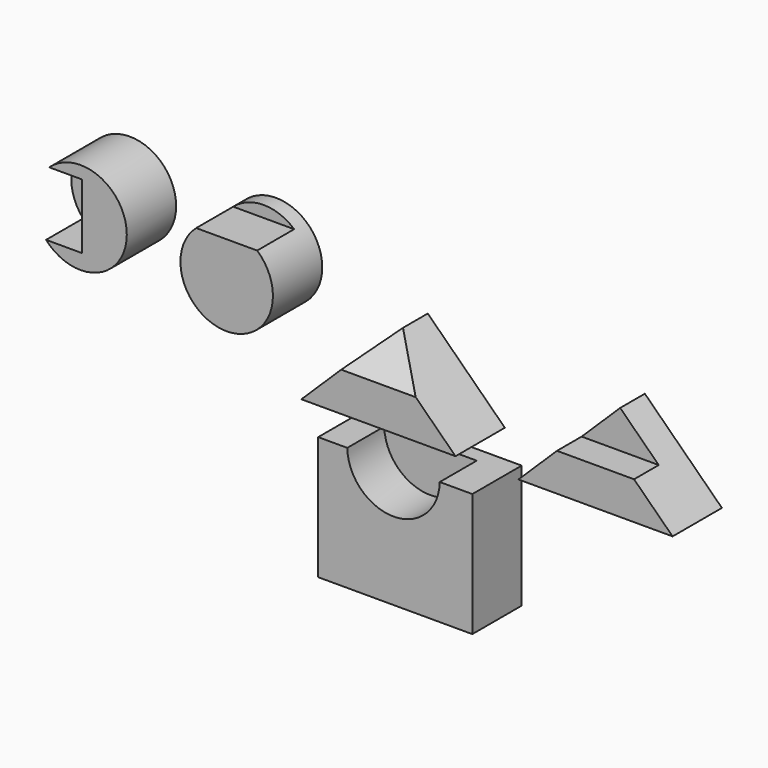
from build123d import *

# Parameters (mm, degrees)
F1_DEPTH  = 101.6
F2_DEPTH  = 50.8
F4_DEPTH  = 101.6
F8_DEPTH  = 63.5
F9_R      = 76.2
F10_DEPTH = 101.6
F11_W     = 138.8424634933
F11_H     = 72.9273408651
F12_DEPTH = 76.2
F13_R     = 76.2
F14_DEPTH = 101.6
F15_W     = 160.2847576141
F15_H     = 106.856547296
F16_DEPTH = 76.2
F17_W     = 254
F17_H     = 203.2
F18_DEPTH = 101.6
F19_R     = 76.2
F20_DEPTH = 76.2


with BuildPart() as f1:
    # F0 (on Front) → F1 (new body)
    with BuildSketch(Plane.XZ):
        Polygon((63.5, 62.2170394667), (0, 0), (254, 0), (190.5, 62.2170394667), align=None)
    extrude(amount=F1_DEPTH)

    # F0 (on Front) → F2 (join)
    with BuildSketch(Plane.XZ):
        Polygon((63.5, 62.2170394667), (0, 0), (254, 0), (190.5, 62.2170394667), align=None)
        Polygon((127, 124.4340789334), (63.5, 62.2170394667), (190.5, 62.2170394667), align=None)
    extrude(amount=F2_DEPTH)


with BuildPart() as f4:
    # F3 (on Front) → F4 (new body)
    with BuildSketch(Plane.XZ):
        Polygon((-357.6793918375, 0), (-103.6793918375, 0), (-230.6793918375, 124.4340789334), align=None)
    extrude(amount=F4_DEPTH)

    # F7 (on 3pt) → F8 (cut, symmetric)
    with BuildSketch(Plane.YZ.offset(-230.6793918375)):
        Polygon((-101.8185078442, 64.035332354), (-51.0185078442, 124.4698180237), (-101.8185078442, 124.4698180237), align=None)
    extrude(amount=F8_DEPTH, both=True, mode=Mode.SUBTRACT)


with BuildPart() as f10:
    # F9 (on Front) → F10 (new body)
    with BuildSketch(Plane.XZ):
        with Locations((-562.0247125626, 66.992148757)):
            Circle(F9_R)
    extrude(amount=-F10_DEPTH)

    # F11 (on Front) → F12 (cut)
    with BuildSketch(Plane.XZ):
        with Locations((-563.4106993675, 160.768315196)):
            Rectangle(F11_W, F11_H)
    extrude(amount=-F12_DEPTH, mode=Mode.SUBTRACT)


with BuildPart() as f14:
    # F13 (on Front) → F14 (new body)
    with BuildSketch(Plane.XZ):
        with Locations((-802.8185963631, 77.5676518679)):
            Circle(F13_R)
    extrude(amount=-F14_DEPTH)

    # F15 (on Front) → F16 (cut)
    with BuildSketch(Plane.XZ):
        with Locations((-880.1847100258, 80.1907256246)):
            Rectangle(F15_W, F15_H)
    extrude(amount=-F16_DEPTH, mode=Mode.SUBTRACT)


with BuildPart() as f18:
    # F17 (on Front) → F18 (new body)
    with BuildSketch(Plane.XZ):
        with Locations((-284.2599749565, -215.2100077792)):
            Rectangle(F17_W, F17_H)
    extrude(amount=-F18_DEPTH)

    # F19 (on Front) → F20 (cut)
    with BuildSketch(Plane.XZ):
        with Locations((-287.1308624744, -112.2424378991)):
            Circle(F19_R)
    extrude(amount=-F20_DEPTH, mode=Mode.SUBTRACT)


solid = Compound([f1.part, f4.part, f10.part, f14.part, f18.part])
